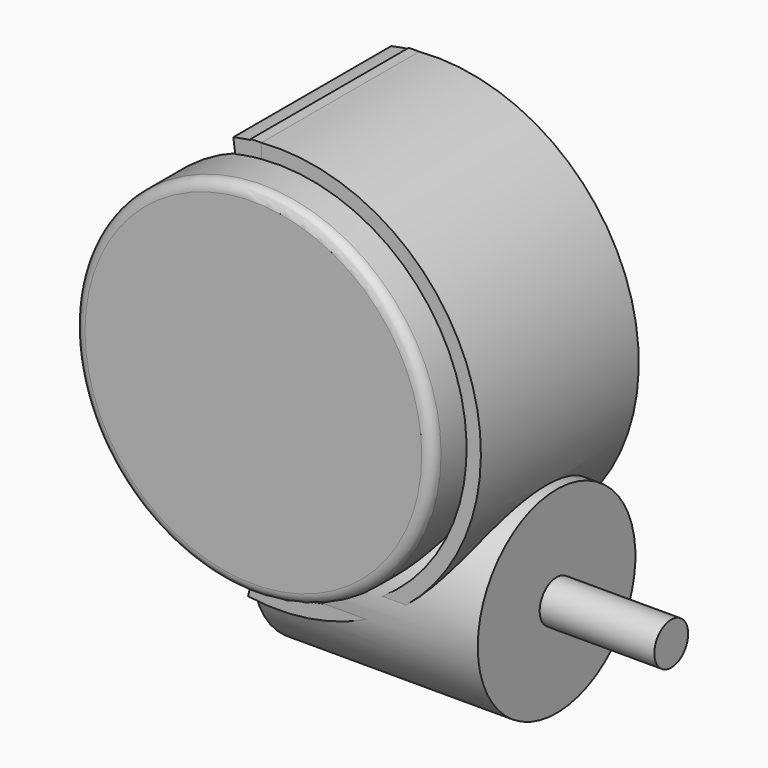
from build123d import *
from build123d import SkipClean  # not in build123d's __all__

# Parameters (mm, degrees)
F0_R      = 4
F1_DEPTH  = 12.7
F2_R      = 31.75
F3_DEPTH  = 10
F4_R      = 1.905
F6_W      = 15.24
F6_H      = 6.6250320524
F7_DEPTH  = 71.12
F9_W      = 1.8474994206
F9_H      = 34.9828377366
F10_DEPTH = 2.54
F11_ANGLE = 8
F12_ANGLE = 193
F13_R     = 3.75
F14_DEPTH = 20.32
F15_R     = 17.4624022324
F16_DEPTH = 40


with BuildPart() as f1:
    # F0 (on Front) → F1 (new body)
    with BuildSketch(Plane.XZ):
        with Locations((-55.9084378183, 37.7567484975)):
            Circle(F0_R)
    extrude(amount=F1_DEPTH)

    # F2 (on face) → F3 (join)
    with BuildSketch(Plane.XZ.offset(12.7)):
        with Locations((-55.9084378183, 37.7567484975)):
            Circle(F2_R)
    extrude(amount=F3_DEPTH)

    # F4
    f4_edges = [f1.edges().sort_by_distance(p)[0] for p in [
        (-87.658438, -22.7, 37.756748),
    ]]
    fillet(f4_edges, radius=F4_R)

    # F5: F1 across plane


with BuildPart() as f1_1:
    add(f1.part, clean=False)
    add(f1.part.mirror(Plane.XZ), clean=False)

    # F6 (on Top) → F7 (join)
    with BuildSketch(Plane.XY):
        with Locations((-53.0349581492, 3.3125160262)):
            Rectangle(F6_W, F6_H)
    extrude(amount=F7_DEPTH)

    # F8: F1 across plane


with BuildPart() as f1_2:
    add(f1_1.part, clean=False)
    add(f1_1.part.mirror(Plane.XZ), clean=False)

    # F9 (on face) → F10 (join)
    with BuildSketch(Plane.XY.offset(71.12)):
        with Locations((-59.7312084389, 0.1775659621)):
            Rectangle(F9_W, F9_H)
    extrude(amount=F10_DEPTH)

    # F10_face (on face) → F11 (revolve)
    with BuildSketch(Plane(origin=(-58.8074587286, 0.1775659621, 72.39), x_dir=(0, 1, 0), z_dir=(1, 0, 0))):
        Polygon((-17.4914188683, 1.27), (-17.4914188683, -1.27), (-6.8025980145, -1.27), (6.4474660903, -1.27), (17.4914188683, -1.27), (17.4914188683, 1.27), align=None)
    revolve(axis=Axis((-55.9084378183, -22.7, 37.7567484975), (0, -1, 0)), revolution_arc=F11_ANGLE)

    # F10_face (on face) → F12 (revolve)
    with BuildSketch(Plane(origin=(-58.8074587286, 0.1775659621, 72.39), x_dir=(0, 1, 0), z_dir=(1, 0, 0))):
        Polygon((-17.4914188683, 1.27), (-17.4914188683, -1.27), (-6.8025980145, -1.27), (6.4474660903, -1.27), (17.4914188683, -1.27), (17.4914188683, 1.27), align=None)
    with SkipClean():  # cleaning this boolean's faces spoils the solid; the shape is the same uncleaned
        revolve(axis=Axis((-55.9084378183, -22.7, 37.7567484975), (0, 1, 0)), revolution_arc=F12_ANGLE)



with BuildPart() as f14:
    # F13 (on Right) → F14 (new body)
    with BuildSketch(Plane.YZ):
        with Locations((0, 7.5903639288)):
            Circle(F13_R)
    extrude(amount=-F14_DEPTH)


with BuildPart() as f1_3:
    add(f1_2.part, clean=False)

    with SkipClean():  # cleaning this boolean's faces spoils the solid; the shape is the same uncleaned
        add(f14.part)  # F16 merges F14
    # F15 (on face) → F16 (join)
    with BuildSketch(Plane(origin=(-20.32, 0, 0), x_dir=(0, -1, 0), z_dir=(-1, 0, 0))):
        with Locations((0, 7.5903639288)):
            Circle(F15_R)
    with SkipClean():  # cleaning this boolean's faces spoils the solid; the shape is the same uncleaned
        extrude(amount=F16_DEPTH)


solid = f1_3.part
